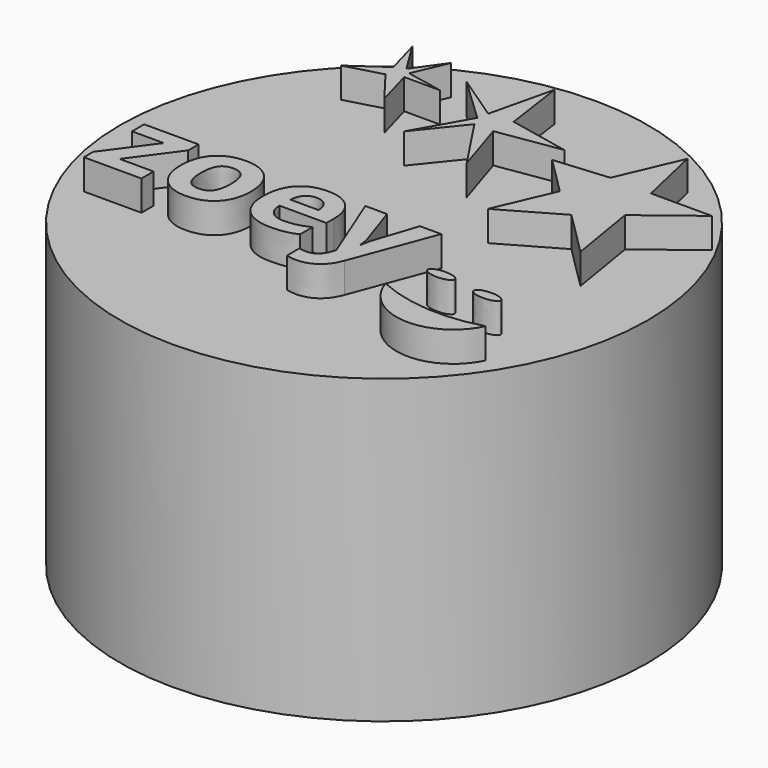
from build123d import *

# Parameters (mm, degrees)
F0_R         = 17.5
F1_DEPTH     = 20
F3_DEPTH     = 2
F2_TEXT_SIZE = 8.8527320056
F4_DEPTH     = 2
F5_DEPTH     = 2


# Not quite as in the source:
# - Text() gives the source's letters only with a copy of the font that has no kerning and outlines rounded to 1/6400 em; it was checked with that copy


with BuildPart() as f1:
    # F0 (on Top) → F1 (new body)
    with BuildSketch(Plane.XY):
        Circle(F0_R)
    extrude(amount=F1_DEPTH)

    # F2 (on face) → F3 (join)
    with BuildSketch(Plane.XY.offset(20)):
        Polygon((-8.7857026357, 13.3235421928), (-8.1169067847, 10.9213415497), (-10.3384141112, 9.3653173351), (-7.9291746646, 10.036072857), (-6.275477066, 7.8719990755), (-6.9794281626, 10.4004713655), (-4.5927705334, 10.4004713655), (-7.0388924825, 10.8836593004), (-6.0683592638, 13.1582068053), (-7.4722653608, 11.1930615268), align=None)
    extrude(amount=F3_DEPTH)

    # F2 (on face) → F4 (join)
    with BuildSketch(Plane.XY.offset(20)):
        Polygon((-0.0119141704, 14.1439976764), (-1.0189398603, 9.9065297958), (-4.1552938435, 12.0250256282), (-1.1687142663, 9.1918115528), (-3.1859104384, 5.6301559946), (-0.8420405849, 8.5402763345), (1.5682747598, 4.8968213125), (0.4081586192, 8.5402763345), (4.6095080315, 9.1918115528), (0.5741831099, 10.0243887563), align=None)
        Polygon((10.1894158212, 12.3947826268), (8.4058782086, 8.2535552792), (4.8036008534, 7.9296077602), (7.3046660042, 5.4395120625), (5.6374920532, 1.5684715472), (9.429935911, 3.7416506622), (12.3817538843, 0.8027791046), (11.6160297766, 5.4558324628), (15.1795903221, 8.1946547143), (11.1448140815, 8.1946547143), align=None)
        with Locations((-14.5528346766, -6.9799424382)):
            Text('zoey', F2_TEXT_SIZE, font='Open Sans', font_style=FontStyle.BOLD, text_align=(TextAlign.LEFT, TextAlign.BOTTOM))
    extrude(amount=F4_DEPTH)

    # F2 (on face) → F5 (join)
    with BuildSketch(Plane.XY.offset(20)):
        with BuildLine():
            ThreePointArc((13.7587697245, -8.7732793763), (10.1979233323, -9.1552375477), (6.7257531919, -8.2779955119))
            ThreePointArc((6.7257531919, -8.2779955119), (10.0723528073, -10.9383353671), (13.7587697245, -8.7732793763))
        make_face()
        with BuildLine():
            add(Edge.make_bspline(
                [(7.4544791132, -5.6871259585), (7.4544791132, -6.3073188332), (8.791743312, -5.9972223958), (10.1290075108, -5.6871259585), (8.791743312, -5.3770295212), (7.4544791132, -5.0669330838), (7.4544791132, -5.6871259585)],
                knots=[0, 0, 0, 2.0943951024, 2.0943951024, 4.1887902048, 4.1887902048, 6.2831853072, 6.2831853072, 6.2831853072], degree=2, weights=[1, 0.5, 1, 0.5, 1, 0.5, 1]))
        make_face()
        with BuildLine():
            add(Edge.make_bspline(
                [(10.7807255195, -6.0312914045), (10.7807255195, -6.6514842791), (12.1179897183, -6.3413878418), (13.4552539171, -6.0312914045), (12.1179897183, -5.7211949671), (10.7807255195, -5.4110985298), (10.7807255195, -6.0312914045)],
                knots=[0, 0, 0, 2.0943951024, 2.0943951024, 4.1887902048, 4.1887902048, 6.2831853072, 6.2831853072, 6.2831853072], degree=2, weights=[1, 0.5, 1, 0.5, 1, 0.5, 1]))
        make_face()
    extrude(amount=F5_DEPTH)


solid = f1.part
